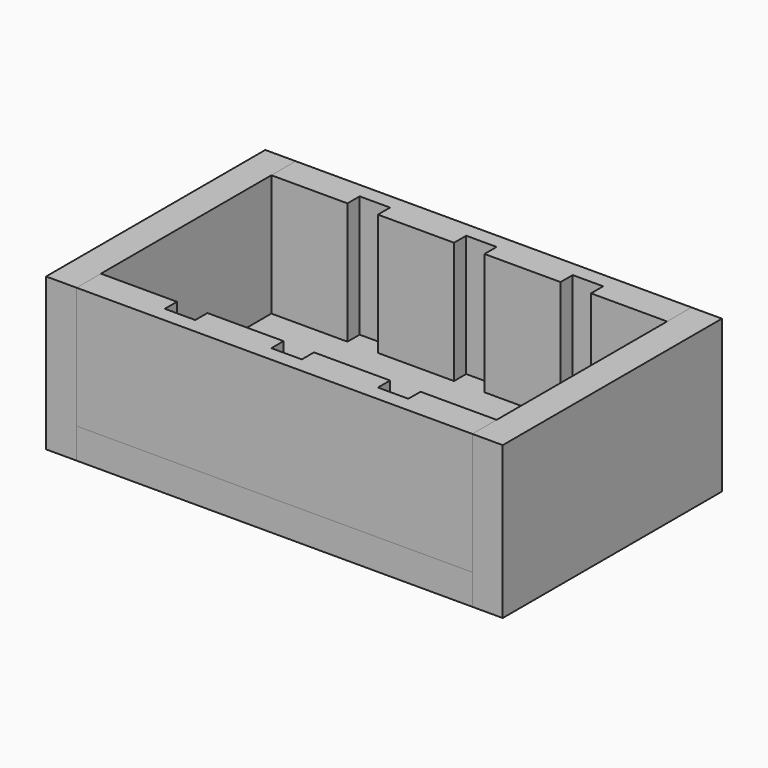
from build123d import *

# Parameters (mm, degrees)
F2_W      = 165.1
F2_H      = 50.8
F3_DEPTH  = 12.7
F0_W      = 165.1
F0_H      = 114.3
F4_DEPTH  = 12.7
F6_W      = 165.1
F6_H      = 50.8
F7_DEPTH  = 12.7
F9_W      = 88.9
F9_H      = 50.8
F9_W_2    = 12.7
F10_DEPTH = 12.7
F12_W     = 88.9
F12_H     = 50.8
F12_W_2   = 12.7
F13_DEPTH = 12.7
F14_W     = 12.7
F14_H     = 6.35
F15_DEPTH = 63.5
F16_W     = 12.7
F16_H     = 6.35
F17_DEPTH = 63.5


with BuildPart() as f3:
    # F2 (on line) → F3 (new body)
    with BuildSketch(Plane(origin=(0, 57.15, 0), x_dir=(-1, 0, 0), z_dir=(0, 1, 0))):
        with Locations((0, 25.4)):
            Rectangle(F2_W, F2_H)
    extrude(amount=-F3_DEPTH)

    # F14 (on face) → F15 (cut)
    with BuildSketch(Plane.XY.offset(50.8)):
        with Locations((-44.45, 47.625)):
            Rectangle(F14_W, F14_H)
        with Locations((0, 47.625)):
            Rectangle(F14_W, F14_H)
        with Locations((44.45, 47.625)):
            Rectangle(F14_W, F14_H)
    extrude(amount=-F15_DEPTH, mode=Mode.SUBTRACT)


with BuildPart() as f4:
    # F0 (on Top) → F4 (new body)
    with BuildSketch(Plane.XY):
        Rectangle(F0_W, F0_H)
    extrude(amount=-F4_DEPTH)


with BuildPart() as f7:
    # F6 (on face) → F7 (new body)
    with BuildSketch(Plane(origin=(0, -57.15, 0), x_dir=(-1, 0, 0), z_dir=(0, 1, 0))):
        with Locations((0, 25.4)):
            Rectangle(F6_W, F6_H)
    extrude(amount=F7_DEPTH)

    # F16 (on face) → F17 (cut)
    with BuildSketch(Plane.XY.offset(50.8)):
        with Locations((44.45, -47.625)):
            Rectangle(F16_W, F16_H)
        with Locations((0, -47.625)):
            Rectangle(F16_W, F16_H)
        with Locations((-44.45, -47.625)):
            Rectangle(F16_W, F16_H)
    extrude(amount=-F17_DEPTH, mode=Mode.SUBTRACT)


with BuildPart() as f10:
    # F9 (on face) → F10 (new body)
    with BuildSketch(Plane(origin=(82.55, 0, 0), x_dir=(0, -1, 0), z_dir=(-1, 0, 0))):
        with Locations((0, 25.4)):
            Rectangle(F9_W, F9_H)
        with Locations((50.8, 25.4)):
            Rectangle(F9_W_2, F9_H)
        with Locations((-50.8, 25.4)):
            Rectangle(F9_W_2, F9_H)
        Polygon((57.15, -12.7), (57.15, 0), (44.45, 0), (-44.45, 0), (-57.15, 0), (-57.15, -12.7), align=None)
    extrude(amount=-F10_DEPTH)


with BuildPart() as f13:
    # F12 (on face) → F13 (new body)
    with BuildSketch(Plane(origin=(-82.55, 0, 0), x_dir=(0, -1, 0), z_dir=(-1, 0, 0))):
        with Locations((0, 25.4)):
            Rectangle(F12_W, F12_H)
        with Locations((50.8, 25.4)):
            Rectangle(F12_W_2, F12_H)
        Polygon((-44.45, 0), (-57.15, 0), (-57.15, -12.7), (57.15, -12.7), (57.15, 0), (44.45, 0), align=None)
        with Locations((-50.8, 25.4)):
            Rectangle(F12_W_2, F12_H)
    extrude(amount=F13_DEPTH)


solid = Compound([f3.part, f4.part, f7.part, f10.part, f13.part])
